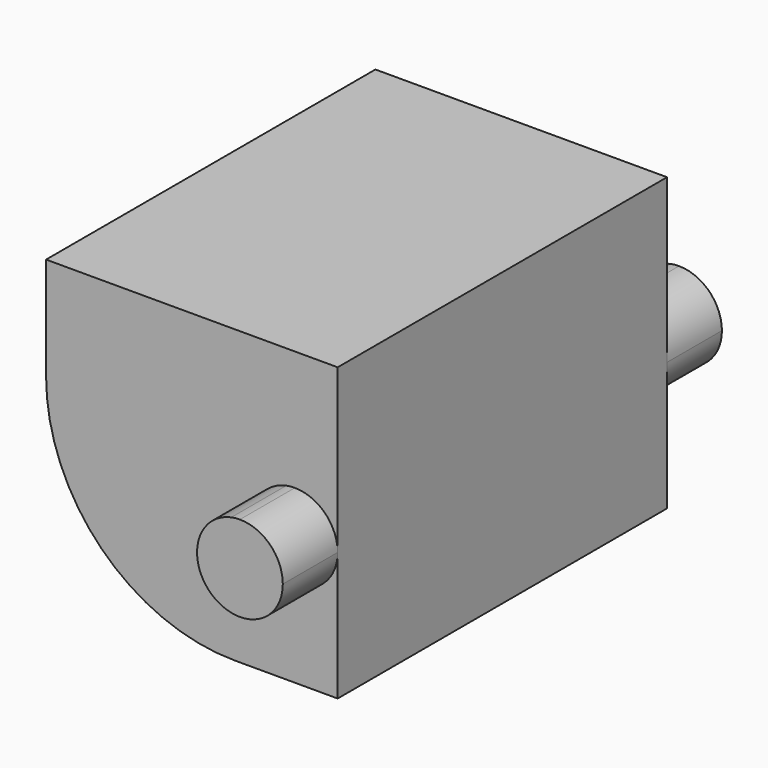
from build123d import *

# Parameters (mm, degrees)
F0_W     = 14
F0_H     = 12
F1_DEPTH = 24
F3_DEPTH = 28
F4_DEPTH = 4
F6_DEPTH = 24
F8_DEPTH = 24
F9_R     = 11


with BuildPart() as f1:
    # F0 (on Front) → F1 (new body)
    with BuildSketch(Plane.XZ):
        with Locations((-47.7052051574, 17.2259079414)):
            Rectangle(F0_W, F0_H)
    extrude(amount=F1_DEPTH)

    # F2 (on face) → F3 (join)
    with BuildSketch(Plane.XZ.offset(24)):
        with BuildLine():
            ThreePointArc((-40.7052051574, 11.2764181987), (-40.4564775624, 11.2385675589), (-40.2052051574, 11.2259079414))
            ThreePointArc((-40.2052051574, 11.2259079414), (-38.4374382044, 11.9581409885), (-37.7052051574, 13.7259079414))
            ThreePointArc((-37.7052051574, 13.7259079414), (-38.4374382044, 15.4936748944), (-40.2052051574, 16.2259079414))
            ThreePointArc((-40.2052051574, 16.2259079414), (-40.4564775624, 16.2132483239), (-40.7052051574, 16.1753976842))
            Line((-40.7052051574, 16.1753976842), (-40.7052051574, 11.2764181987))
        make_face()
        with BuildLine():
            ThreePointArc((-40.7052051574, 16.1753976842), (-42.7052051574, 13.7259079414), (-40.7052051574, 11.2764181987))
            Line((-40.7052051574, 11.2764181987), (-40.7052051574, 16.1753976842))
        make_face()
    extrude(amount=-F3_DEPTH)

    # F2 (on face) → F4 (join)
    with BuildSketch(Plane.XZ.offset(24)):
        with BuildLine():
            ThreePointArc((-40.7052051574, 11.2764181987), (-40.4564775624, 11.2385675589), (-40.2052051574, 11.2259079414))
            ThreePointArc((-40.2052051574, 11.2259079414), (-38.4374382044, 11.9581409885), (-37.7052051574, 13.7259079414))
            ThreePointArc((-37.7052051574, 13.7259079414), (-38.4374382044, 15.4936748944), (-40.2052051574, 16.2259079414))
            ThreePointArc((-40.2052051574, 16.2259079414), (-40.4564775624, 16.2132483239), (-40.7052051574, 16.1753976842))
            Line((-40.7052051574, 16.1753976842), (-40.7052051574, 11.2764181987))
        make_face()
        with BuildLine():
            ThreePointArc((-40.7052051574, 16.1753976842), (-42.7052051574, 13.7259079414), (-40.7052051574, 11.2764181987))
            Line((-40.7052051574, 11.2764181987), (-40.7052051574, 16.1753976842))
        make_face()
    extrude(amount=F4_DEPTH)

    # F5 (on face) → F6 (join)
    with BuildSketch(Plane.XZ.offset(24)):
        Polygon((-37.7052051574, 23.2259079414), (-40.7052051574, 23.2259079414), (-40.7052051574, 16.1753976842), (-40.7052051574, 13.2259079414), (-37.7052051574, 13.2259079414), align=None)
    extrude(amount=-F6_DEPTH)

    # F7 (on face) → F8 (join)
    with BuildSketch(Plane.XZ.offset(24)):
        with BuildLine():
            Line((-40.7052051574, 11.2259079414), (-54.7052051574, 11.2259079414))
            Line((-54.7052051574, 11.2259079414), (-54.7052051574, 6.2259079414))
            Line((-54.7052051574, 6.2259079414), (-37.7052051574, 6.2259079414))
            Line((-37.7052051574, 6.2259079414), (-37.7052051574, 13.2259079414))
            Line((-37.7052051574, 13.2259079414), (-37.7557154146, 13.2259079414))
            ThreePointArc((-37.7557154146, 13.2259079414), (-37.7178647749, 13.4746355364), (-37.7052051574, 13.7259079414))
            ThreePointArc((-37.7052051574, 13.7259079414), (-41.7863439875, 15.6623996145), (-40.7052051574, 11.2764181987))
            Line((-40.7052051574, 11.2764181987), (-40.7052051574, 11.2259079414))
        make_face()
    extrude(amount=-F8_DEPTH)

    # F9
    f9_edges = [f1.edges().sort_by_distance(p)[0] for p in [
        (-54.705205, -12, 6.225908),
    ]]
    fillet(f9_edges, radius=F9_R)


solid = f1.part
